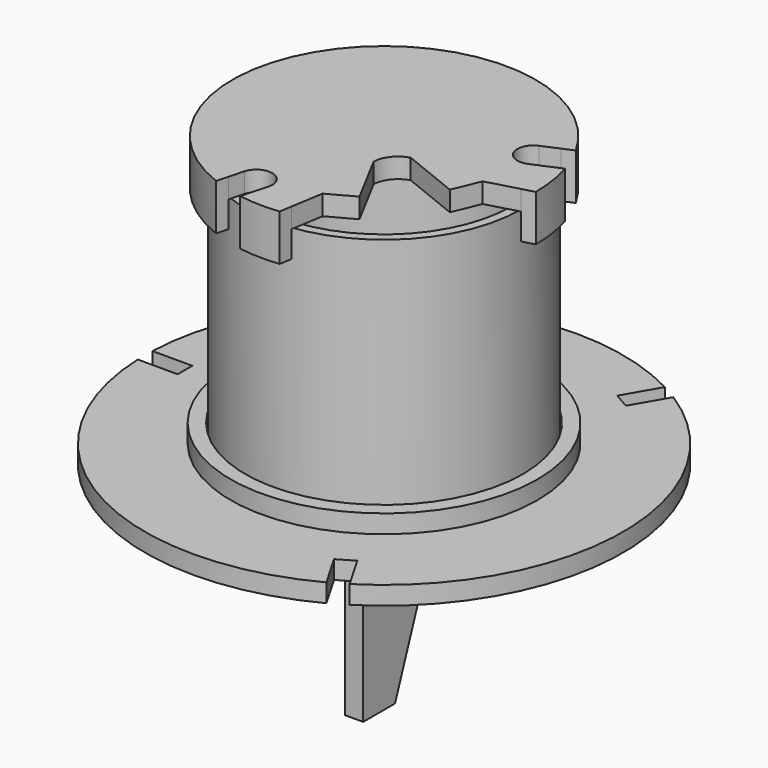
from build123d import *

# Parameters (mm, degrees)
F0_R      = 43.815
F0_R_2    = 40.9575
F1_DEPTH  = 79.9846
F2_W      = 40.64
F2_H      = 40.64
F3_DEPTH  = 5.842
F4_DEPTH  = 5.843
F6_DEPTH  = 5.842
F8_DEPTH  = 8.382
F9_DEPTH  = 6.35
F0_R_3    = 48.895
F0_R_4    = 44.2976
F10_DEPTH = 5.842
F11_DEPTH = 1.27


# Not quite as in the source:
# - a feature names something its author has since deleted; it is built from what else it names


with BuildPart() as f1:
    # F0 (on Top) → F1 (new body)
    with BuildSketch(Plane.XY):
        Circle(F0_R)
        Circle(F0_R_2, mode=Mode.SUBTRACT)
    extrude(amount=F1_DEPTH)

    # F2 (on Top) → F4 (cut, through all)
    with BuildSketch(Plane.XY):
        Rectangle(F2_W, F2_H)
    extrude(amount=-F4_DEPTH, mode=Mode.SUBTRACT)


with BuildPart() as f3:
    # F2 (on Top) → F3 (new body)
    with BuildSketch(Plane.XY):
        with BuildLine():
            Line((-63.4439935845, -2.921), (-76.1439935845, -2.921))
            ThreePointArc((-76.1439935845, -2.921), (-38.1, -65.9911357684), (35.5423365878, -67.4031327898))
            Line((35.5423365878, -67.4031327898), (29.1923365878, -56.4046101617))
            Line((29.1923365878, -56.4046101617), (34.2516569967, -53.4836101617))
            Line((34.2516569967, -53.4836101617), (40.6016569967, -64.4821327898))
            ThreePointArc((40.6016569967, -64.4821327898), (76.2, 0), (40.6016569967, 64.4821327898))
            Line((40.6016569967, 64.4821327898), (34.2516569967, 53.4836101617))
            Line((34.2516569967, 53.4836101617), (29.1923365878, 56.4046101617))
            Line((29.1923365878, 56.4046101617), (35.5423365878, 67.4031327898))
            ThreePointArc((35.5423365878, 67.4031327898), (-38.1, 65.9911357684), (-76.1439935845, 2.921))
            Line((-76.1439935845, 2.921), (-63.4439935845, 2.921))
            Line((-63.4439935845, 2.921), (-63.4439935845, -2.921))
        make_face()
        Rectangle(F2_W, F2_H, mode=Mode.SUBTRACT)
    extrude(amount=-F3_DEPTH)

    # F0 (on Top) → F11 (cut)
    with BuildSketch(Plane.XY):
        Circle(F0_R_3)
        Circle(F0_R_4, mode=Mode.SUBTRACT)
    extrude(amount=-F11_DEPTH, mode=Mode.SUBTRACT)


with BuildPart() as f6:
    # F5 (on Right) → F6 (new body)
    with BuildSketch(Plane.YZ):
        with BuildLine():
            Line((-15.621, -69.85), (-2.921, -69.85))
            Line((-2.921, -69.85), (16.1294304292, -19.0553526104))
            ThreePointArc((16.1294304292, -19.0553526104), (20.6192802377, -17.1953285033), (22.479, -12.705352625))
            Line((22.479, -12.705352625), (22.479, -5.6642))
            Line((22.479, -5.6642), (9.779, -5.6642))
            Line((9.779, -5.6642), (9.779, 0))
            Line((9.779, 0), (22.479, 0))
            Line((22.479, 0), (22.479, 5.08))
            ThreePointArc((22.479, 5.08), (20.2471536726, 10.4681536726), (14.859, 12.7))
            Line((14.859, 12.7), (-8.001, 12.7))
            ThreePointArc((-8.001, 12.7), (-13.3891536726, 10.4681536726), (-15.621, 5.08))
            Line((-15.621, 5.08), (-15.621, -69.85))
        make_face()
    extrude(amount=F6_DEPTH)


with BuildPart() as f8:
    # F7 (on face) → F8 (new body)
    with BuildSketch(Plane.XY.offset(79.9846)):
        with BuildLine():
            ThreePointArc((42.675855879, 12.7912621565), (44.1536785796, 5.9411893128), (44.5390860822, -1.0558757115))
            Line((44.5390860822, -1.0558757115), (48.3616, 0))
            ThreePointArc((48.3616, 0), (47.8176579237, 7.2329762373), (46.198067559, 14.3032481757))
            Line((46.198067559, 14.3032481757), (42.675855879, 12.7912621565))
        make_face()
    extrude(amount=-F8_DEPTH)



with BuildPart() as f8b:
    # F7 (on face) → F8, piece 2 (new body)
    with BuildSketch(Plane.XY.offset(79.9846)):
        with BuildLine():
            Line((5.1829115282, -48.0830716849), (5.8230474227, -44.1694145453))
            ThreePointArc((5.8230474227, -44.1694145453), (-0.4201112399, -44.5496191803), (-6.6549894488, -44.0517443241))
            Line((-6.6549894488, -44.0517443241), (-7.6559784913, -47.7517575373))
            ThreePointArc((-7.6559784913, -47.7517575373), (-1.2475805854, -48.3455054503), (5.1829115282, -48.0830716849))
        make_face()
    extrude(amount=-F8_DEPTH)


with BuildPart() as f8c:
    # F7 (on face) → F8, piece 3 (new body)
    with BuildSketch(Plane.XY.offset(79.9846)):
        with BuildLine():
            ThreePointArc((-16.4624232954, -41.3984743898), (-33.6475489603, 29.2008135422), (38.6681126614, 22.127406666))
            Line((38.6681126614, 22.127406666), (42.1903243414, 23.6393926852))
            ThreePointArc((42.1903243414, 23.6393926852), (-36.525047446, 31.6980324882), (-17.4634123379, -45.098487603))
            Line((-17.4634123379, -45.098487603), (-16.4624232954, -41.3984743898))
        make_face()
    extrude(amount=-F8_DEPTH)


with BuildPart() as f8_1:
    add(f8.part)

    add(f8b.part)  # F9 merges F8b

    add(f8c.part)  # F9 merges F8c
    # F7 (on face) → F9 (join)
    with BuildSketch(Plane.XY.offset(79.9846)):
        with BuildLine():
            Line((34.489602072, -3.8317991766), (44.5390860822, -1.0558757115))
            ThreePointArc((44.5390860822, -1.0558757115), (44.1536785796, 5.9411893128), (42.675855879, 12.7912621565))
            Line((42.675855879, 12.7912621565), (37.4123476678, 10.5317867047))
            ThreePointArc((37.4123476678, 10.5317867047), (30.7404038042, 13.1959873507), (33.4046044502, 19.8679312142))
            Line((33.4046044502, 19.8679312142), (38.6681126614, 22.127406666))
            ThreePointArc((38.6681126614, 22.127406666), (-33.6475489603, 29.2008135422), (-16.4624232954, -41.3984743898))
            Line((-16.4624232954, -41.3984743898), (-15.1854641746, -36.6783771467))
            ThreePointArc((-15.1854641746, -36.6783771467), (-8.9551122842, -33.1012951905), (-5.378030328, -39.331647081))
            Line((-5.378030328, -39.331647081), (-6.6549894488, -44.0517443241))
            ThreePointArc((-6.6549894488, -44.0517443241), (-0.4201112399, -44.5496191803), (5.8230474227, -44.1694145453))
            Line((5.8230474227, -44.1694145453), (7.5059805853, -33.8803127415))
            Line((7.5059805853, -33.8803127415), (15.690090875, -29.4144514582))
            Line((15.690090875, -29.4144514582), (6.6396118432, -12.4473810776))
            ThreePointArc((6.6396118432, -12.4473810776), (8.394602452, -7.7932588029), (12.5425105212, -5.0481349743))
            Line((12.5425105212, -5.0481349743), (30.9265518698, -12.4473810776))
            Line((30.9265518698, -12.4473810776), (34.489602072, -3.8317991766))
        make_face()
        with BuildLine():
            ThreePointArc((42.675855879, 12.7912621565), (44.1536785796, 5.9411893128), (44.5390860822, -1.0558757115))
            Line((44.5390860822, -1.0558757115), (48.3616, 0))
            ThreePointArc((48.3616, 0), (47.8176579237, 7.2329762373), (46.198067559, 14.3032481757))
            Line((46.198067559, 14.3032481757), (42.675855879, 12.7912621565))
        make_face()
        with BuildLine():
            ThreePointArc((-16.4624232954, -41.3984743898), (-33.6475489603, 29.2008135422), (38.6681126614, 22.127406666))
            Line((38.6681126614, 22.127406666), (42.1903243414, 23.6393926852))
            ThreePointArc((42.1903243414, 23.6393926852), (-36.525047446, 31.6980324882), (-17.4634123379, -45.098487603))
            Line((-17.4634123379, -45.098487603), (-16.4624232954, -41.3984743898))
        make_face()
        with BuildLine():
            Line((5.1829115282, -48.0830716849), (5.8230474227, -44.1694145453))
            ThreePointArc((5.8230474227, -44.1694145453), (-0.4201112399, -44.5496191803), (-6.6549894488, -44.0517443241))
            Line((-6.6549894488, -44.0517443241), (-7.6559784913, -47.7517575373))
            ThreePointArc((-7.6559784913, -47.7517575373), (-1.2475805854, -48.3455054503), (5.1829115282, -48.0830716849))
        make_face()
    extrude(amount=F9_DEPTH)


with BuildPart() as f10:
    # F0 (on Top) → F10 (new body)
    with BuildSketch(Plane.XY):
        Circle(F0_R_3)
        Circle(F0_R_4, mode=Mode.SUBTRACT)
    extrude(amount=F10_DEPTH)


solid = Compound([f1.part, f3.part, f6.part, f8_1.part, f10.part])
